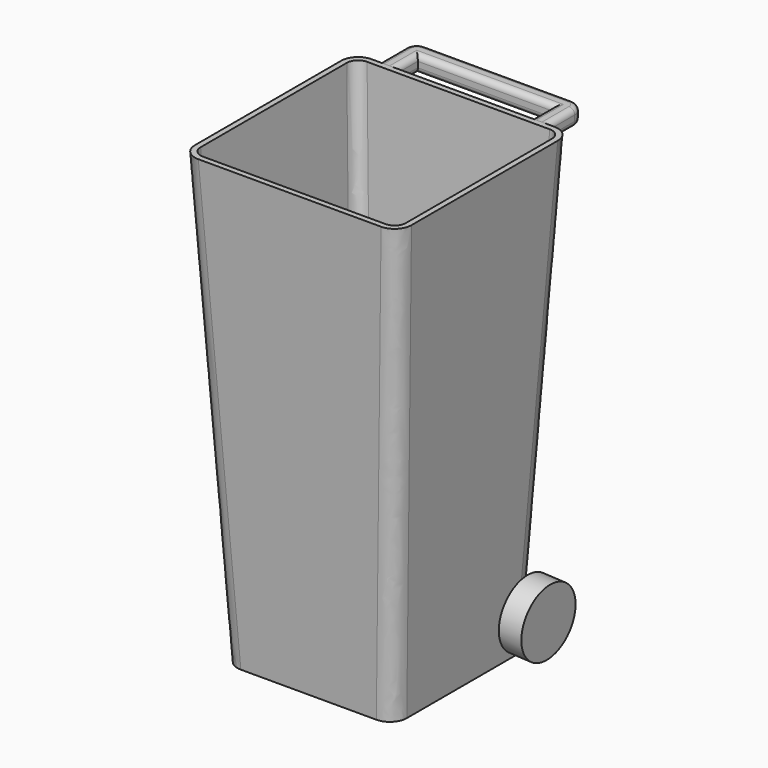
from build123d import *

# Parameters (mm, degrees)
F0_W     = 381
F0_H     = 381
F1_DEPTH = 1016
F1_TAPER = -3
F3_DEPTH = 38.1
F4_R     = 76.2
F5_DEPTH = 50.8
F7_R     = 38.1
F8_T     = -12.7
F9_R     = 12.7


with BuildPart() as f1:
    # F0 (on Top) → F1 (new body)
    with BuildSketch(Plane.XY):
        Rectangle(F0_W, F0_H)
    extrude(amount=F1_DEPTH, taper=F1_TAPER)

    # F7
    f7_edges = [f1.edges().sort_by_distance(p)[0] for p in [
        (217.123152, -217.123152, 508),
        (217.123152, 217.123152, 508),
        (-217.123152, -217.123152, 508),
        (-217.123152, 217.123152, 508),
    ]]
    fillet(f7_edges, radius=F7_R)

    # F8
    f8_openings = [f1.faces().sort_by_distance(p)[0] for p in [
        (0, 0, 1016),
    ]]
    offset(amount=F8_T, openings=f8_openings)


with BuildPart() as f3:
    # F2 (on face) → F3 (new body)
    with BuildSketch(Plane.XY.offset(1016)):
        with BuildLine():
            Line((152.4, 243.7463037516), (190.5, 243.7463037516))
            Line((190.5, 243.7463037516), (190.5, 319.9463037516))
            ThreePointArc((190.5, 319.9463037516), (183.0605122421, 337.9068159937), (165.1, 345.3463037516))
            Line((165.1, 345.3463037516), (-165.1, 345.3463037516))
            ThreePointArc((-165.1, 345.3463037516), (-183.0605122421, 337.9068159937), (-190.5, 319.9463037516))
            Line((-190.5, 319.9463037516), (-190.5, 243.7463037516))
            Line((-190.5, 243.7463037516), (-152.4, 243.7463037516))
            Line((-152.4, 243.7463037516), (-152.4, 307.2463037516))
            Line((-152.4, 307.2463037516), (152.4, 307.2463037516))
            Line((152.4, 307.2463037516), (152.4, 243.7463037516))
        make_face()
    extrude(amount=-F3_DEPTH)

    # F9
    f9_edges = [f3.edges().sort_by_distance(p)[0] for p in [
        (152.4, 275.496304, 1016),
        (0, 307.246304, 1016),
        (-152.4, 275.496304, 1016),
        (-190.5, 281.846304, 1016),
        (-190.5, 281.846304, 977.9),
        (-152.4, 275.496304, 977.9),
        (0, 307.246304, 977.9),
        (152.4, 275.496304, 977.9),
    ]]
    fillet(f9_edges, radius=F9_R)


with BuildPart() as f5:
    # F4 (on face) → F5 (new body)
    with BuildSketch(Plane(origin=(189.9782105338, 0, -9.9563361262), x_dir=(0, 1, 0), z_dir=(0.9986295348, 0, -0.0523359562))):
        with Locations((177.8, 86.1699996643)):
            Circle(F4_R)
    extrude(amount=F5_DEPTH)


with BuildPart() as f6_1:
    # F6: instance of F5
    add(f5.part.mirror(Plane.YZ))


solid = Compound([f1.part, f3.part, f5.part, f6_1.part])
